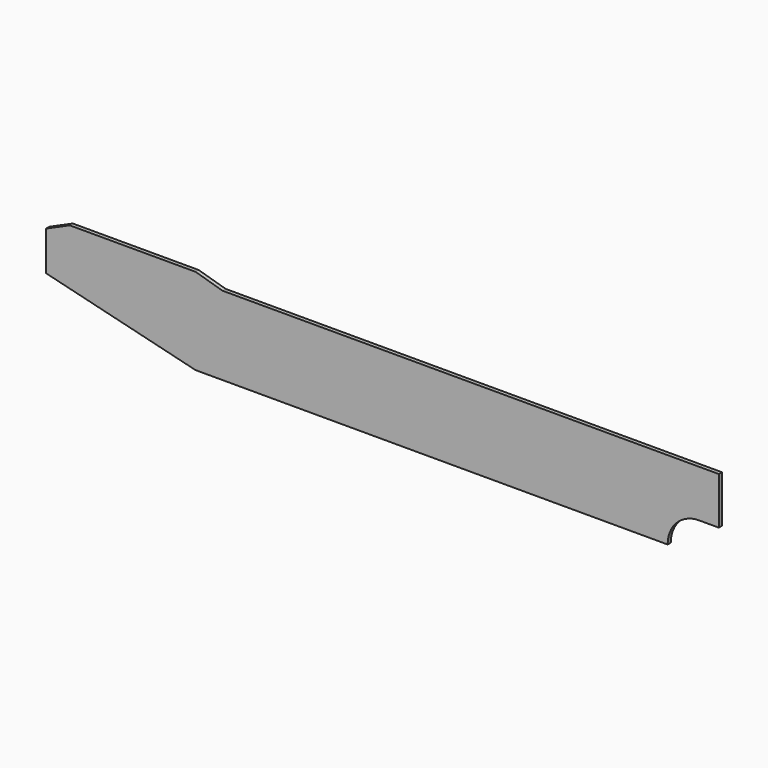
from build123d import *

# Parameters (mm, degrees)
F1_DEPTH = 1.5875


# Not quite as in the source:
# - a length typed as a fraction of an inch, garbled in the dataset ("3 / 203.2 mm" for 3/8 in), is restored


with BuildPart() as f1:
    # F0 (on Front) → F1 (new body)
    with BuildSketch(Plane.XZ):
        with BuildLine():
            Line((-100.4945435773, 16.3548587115), (-100.4945435773, 0.4798587115))
            Line((-100.4945435773, 0.4798587115), (-40.1695435773, -14.3072105065))
            Line((-40.1695435773, -14.3072105065), (150.3304564227, -14.3072105065))
            ThreePointArc((150.3304564227, -14.3072105065), (154.0502003016, -5.3269543854), (163.0304564227, -1.6072105065))
            Line((163.0304564227, -1.6072105065), (170.9679564227, -1.6072105065))
            Line((170.9679564227, -1.6072105065), (170.9679564227, 17.4427894935))
            Line((170.9679564227, 17.4427894935), (-29.290227019, 17.4427894935))
            Line((-29.290227019, 17.4427894935), (-40.1695435773, 20.6177894935))
            Line((-40.1695435773, 20.6177894935), (-90.9695435773, 20.6177894935))
            Line((-90.9695435773, 20.6177894935), (-100.4945435773, 16.3548587115))
        make_face()
    extrude(amount=F1_DEPTH)


solid = f1.part
